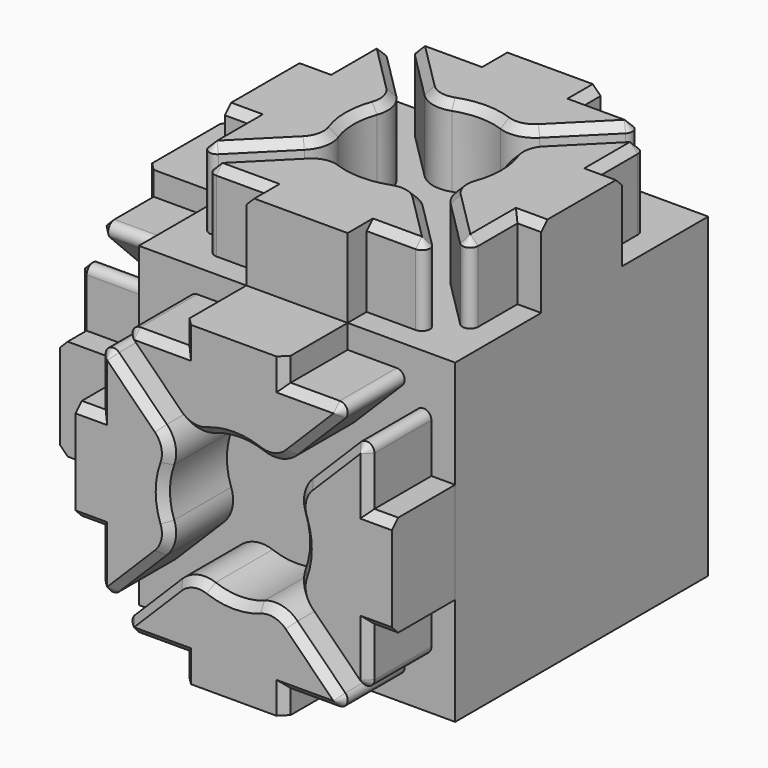
from build123d import *

# Parameters (mm, degrees)
F1_DEPTH     = 5
F3_DEPTH     = 5
F5_DEPTH     = 5
F6_R         = 2.5
F7_DEPTH     = 20
F8_T1_DEPTH  = 8.0177669558
F8_T3_DEPTH  = 8.0177669501
F8_T5_DEPTH  = 8.017766953
F8_T7_DEPTH  = 8.0177669501
F8_T9_DEPTH  = 8.0177669558
F8_T11_DEPTH = 8.0177655359
F8_T13_DEPTH = 8.01776837
F9_R         = 2
F10_SIZE     = 0.49999


# Not quite as in the source:
# - a fillet or chamfer that OpenCascade refuses, or shapes differently, is made with other operations: its cross-section is extruded or revolved along the edge and cut away or added
# - a fillet or chamfer is up to 0.001 mm smaller than in the source, because OpenCascade refuses the exact size


with BuildPart() as f1:
    # F0 (on Top) → F1 (new body)
    with BuildSketch(Plane.XY):
        with BuildLine():
            Line((13.2, 20), (6.8, 20))
            Line((6.8, 20), (6.8, 18.5))
            Line((6.8, 18.5), (2.4899494937, 18.5))
            Line((2.4899494937, 18.5), (7.3899494937, 13.6))
            ThreePointArc((7.3899494937, 13.6), (10, 14.4342618268), (12.6100505063, 13.6))
            Line((12.6100505063, 13.6), (17.5100505063, 18.5))
            Line((17.5100505063, 18.5), (13.2, 18.5))
            Line((13.2, 18.5), (13.2, 20))
        make_face()
    extrude(amount=F1_DEPTH)



with BuildPart() as f1b:
    # F0 (on Top) → F1, piece 2 (new body)
    with BuildSketch(Plane.XY):
        with BuildLine():
            Line((18.5, 6.8), (20, 6.8))
            Line((20, 6.8), (20, 13.2))
            Line((20, 13.2), (18.5, 13.2))
            Line((18.5, 13.2), (18.5, 17.5100505063))
            Line((18.5, 17.5100505063), (13.6, 12.6100505063))
            ThreePointArc((13.6, 12.6100505063), (14.4342618268, 10), (13.6, 7.3899494937))
            Line((13.6, 7.3899494937), (18.5, 2.4899494937))
            Line((18.5, 2.4899494937), (18.5, 6.8))
        make_face()
    extrude(amount=F1_DEPTH)


with BuildPart() as f1c:
    # F0 (on Top) → F1, piece 3 (new body)
    with BuildSketch(Plane.XY):
        with BuildLine():
            Line((6.8, 1.5), (6.8, 0))
            Line((6.8, 0), (13.2, 0))
            Line((13.2, 0), (13.2, 1.5))
            Line((13.2, 1.5), (17.5100505063, 1.5))
            Line((17.5100505063, 1.5), (12.6100505063, 6.4))
            ThreePointArc((12.6100505063, 6.4), (10, 5.5657381732), (7.3899494937, 6.4))
            Line((7.3899494937, 6.4), (2.4899494937, 1.5))
            Line((2.4899494937, 1.5), (6.8, 1.5))
        make_face()
    extrude(amount=F1_DEPTH)

    # F4 (on Front) → F5 (join)
    with BuildSketch(Plane.XZ):
        with BuildLine():
            Line((2.4899494963, -1.5), (7.3899494979, -6.3999999951))
            ThreePointArc((7.3899494979, -6.3999999951), (9.9999827045, -5.5657504858), (12.6100159112, -6.3999999951))
            Line((12.6100159112, -6.3999999951), (17.5100159046, -1.4999999951))
            Line((17.5100159046, -1.4999999951), (13.1999827087, -1.4999999951))
            Line((13.1999827087, -1.4999999951), (13.1999827087, 0))
            Line((13.1999827087, 0), (6.7999827087, 0))
            Line((6.7999827087, 0), (6.7999827087, -1.5))
            Line((6.7999827087, -1.5), (2.4899494963, -1.5))
        make_face()
    extrude(amount=F5_DEPTH)


with BuildPart() as f1d:
    # F0 (on Top) → F1, piece 4 (new body)
    with BuildSketch(Plane.XY):
        with BuildLine():
            Line((1.5, 6.8), (1.5, 2.4899494937))
            Line((1.5, 2.4899494937), (6.4, 7.3899494937))
            ThreePointArc((6.4, 7.3899494937), (5.5657381732, 10), (6.4, 12.6100505063))
            Line((6.4, 12.6100505063), (1.5, 17.5100505063))
            Line((1.5, 17.5100505063), (1.5, 13.2))
            Line((1.5, 13.2), (0, 13.2))
            Line((0, 13.2), (0, 6.8))
            Line((0, 6.8), (1.5, 6.8))
        make_face()
    extrude(amount=F1_DEPTH)

    # F2 (on Right) → F3 (join)
    with BuildSketch(Plane.YZ):
        with BuildLine():
            Line((2.4899734284, -1.5000000049), (7.38997343, -6.4))
            ThreePointArc((7.38997343, -6.4), (10.0000066366, -5.5657504907), (12.6100398432, -6.4))
            Line((12.6100398432, -6.4), (17.5100398367, -1.5))
            Line((17.5100398367, -1.5), (13.1999893277, -1.5))
            Line((13.1999893277, -1.5), (13.1999893277, -4.9e-09))
            Line((13.1999893277, -4.9e-09), (6.8000066408, -4.9e-09))
            Line((6.8000066408, -4.9e-09), (6.8000066408, -1.5000000049))
            Line((6.8000066408, -1.5000000049), (2.4899734284, -1.5000000049))
        make_face()
    extrude(amount=-F3_DEPTH)


with BuildPart() as f3:
    # F2 (on Right) → F3, piece 2 (new body)
    with BuildSketch(Plane.YZ):
        with BuildLine():
            Line((18.5000132602, -2.4899255639), (13.5999893277, -7.3899495029))
            ThreePointArc((13.5999893277, -7.3899495029), (14.4342388275, -9.9999826961), (13.5999893277, -12.6100158894))
            Line((13.5999893277, -12.6100158894), (18.4999893277, -17.5100158829))
            Line((18.4999893277, -17.5100158829), (18.4999893277, -13.1999827003))
            Line((18.4999893277, -13.1999827003), (20.0000066408, -13.1999827003))
            Line((20.0000066408, -13.1999827003), (20.0000132601, -6.8))
            Line((20.0000132601, -6.8), (18.5000132602, -6.8))
            Line((18.5000132602, -6.8), (18.5000132602, -2.4899255639))
        make_face()
    extrude(amount=-F3_DEPTH)


with BuildPart() as f3b:
    # F2 (on Right) → F3, piece 3 (new body)
    with BuildSketch(Plane.YZ):
        with BuildLine():
            ThreePointArc((12.6100571512, -13.5999827003), (10.0000059036, -14.4342445286), (7.38995493, -13.5999818427))
            Line((7.38995493, -13.5999818427), (2.4899499917, -18.499983527))
            Line((2.4899499917, -18.499983527), (6.8000004981, -18.499983527))
            Line((6.8000004981, -18.499983527), (6.8000004981, -19.999983527))
            Line((6.8000004981, -19.999983527), (13.2000004981, -19.9999835137))
            Line((13.2000004981, -19.9999835137), (13.2000004981, -18.4999827003))
            Line((13.2000004981, -18.4999827003), (17.5100571578, -18.4999827003))
            Line((17.5100571578, -18.4999827003), (12.6100571512, -13.5999827003))
        make_face()
    extrude(amount=-F3_DEPTH)


with BuildPart() as f3c:
    # F2 (on Right) → F3, piece 4 (new body)
    with BuildSketch(Plane.YZ):
        with BuildLine():
            Line((1.5000008268, -13.1999827003), (1.5000008268, -17.5100337047))
            Line((1.5000008268, -17.5100337047), (6.4000024537, -12.6100353317))
            ThreePointArc((6.4000024537, -12.6100353317), (5.5657406284, -9.9999825644), (6.4000050789, -7.3899306362))
            Line((6.4000050789, -7.3899306362), (1.5, -2.4899255639))
            Line((1.5, -2.4899255639), (1.5, -6.7999827003))
            Line((1.5, -6.7999827003), (0, -6.7999827003))
            Line((0, -6.7999827003), (6.6408e-06, -13.1999827003))
            Line((6.6408e-06, -13.1999827003), (1.5000008268, -13.1999827003))
        make_face()
    extrude(amount=-F3_DEPTH)

    # F4 (on Front) → F5, piece 4 (join)
    with BuildSketch(Plane.XZ):
        with BuildLine():
            Line((1.4999827087, -13.1999826954), (1.4999827087, -17.5100332017))
            Line((1.4999827087, -17.5100332017), (6.3999827087, -12.6100332017))
            ThreePointArc((6.3999827087, -12.6100332017), (5.5657208833, -9.9999826974), (6.3999827087, -7.3899321932))
            Line((6.3999827087, -7.3899321932), (1.4999760679, -2.4899255589))
            Line((1.4999760679, -2.4899255589), (1.4999760679, -6.7999826954))
            Line((1.4999760679, -6.7999826954), (-2.39321e-05, -6.7999826954))
            Line((-2.39321e-05, -6.7999826954), (-1.72913e-05, -13.1999826954))
            Line((-1.72913e-05, -13.1999826954), (1.4999827087, -13.1999826954))
        make_face()
    extrude(amount=F5_DEPTH)


with BuildPart() as f5:
    # F4 (on Front) → F5, piece 2 (new body)
    with BuildSketch(Plane.XZ):
        with BuildLine():
            Line((18.4999893281, -2.4899255589), (13.5999653956, -7.3899494979))
            ThreePointArc((13.5999653956, -7.3899494979), (14.4342148954, -9.9999826912), (13.5999653956, -12.6100158845))
            Line((13.5999653956, -12.6100158845), (18.4999653956, -17.510015878))
            Line((18.4999653956, -17.510015878), (18.4999653956, -13.1999826954))
            Line((18.4999653956, -13.1999826954), (19.9999827087, -13.1999826954))
            Line((19.9999827087, -13.1999826954), (19.9999893281, -6.7999826954))
            Line((19.9999893281, -6.7999826954), (18.4999893281, -6.7999826954))
            Line((18.4999893281, -6.7999826954), (18.4999893281, -2.4899255589))
        make_face()
    extrude(amount=F5_DEPTH)


with BuildPart() as f5b:
    # F4 (on Front) → F5, piece 3 (new body)
    with BuildSketch(Plane.XZ):
        with BuildLine():
            ThreePointArc((12.6100332192, -13.5999826954), (9.9999827108, -14.4342445236), (7.3899322023, -13.5999826954))
            Line((7.3899322023, -13.5999826954), (2.4899322023, -18.4999826954))
            Line((2.4899322023, -18.4999826954), (6.7999827087, -18.4999826954))
            Line((6.7999827087, -18.4999826954), (6.7999827087, -19.9999826954))
            Line((6.7999827087, -19.9999826954), (13.1999827087, -19.999982682))
            Line((13.1999827087, -19.999982682), (13.1999827087, -18.4999826954))
            Line((13.1999827087, -18.4999826954), (17.5100332257, -18.4999826954))
            Line((17.5100332257, -18.4999826954), (12.6100332192, -13.5999826954))
        make_face()
    extrude(amount=F5_DEPTH)


with BuildPart() as f1_1:
    add(f1.part)

    add(f1b.part)  # F7 merges F1b

    add(f1c.part)  # F7 merges F1c

    add(f1d.part)  # F7 merges F1d

    add(f3.part)  # F7 merges F3

    add(f3b.part)  # F7 merges F3b

    add(f3c.part)  # F7 merges F3c

    add(f5.part)  # F7 merges F5

    add(f5b.part)  # F7 merges F5b
    # F6 (on face) → F7 (join)
    with BuildSketch(Plane.XY):
        with BuildLine():
            Line((0, 6.8), (0, 0))
            Line((0, 0), (6.8, 0))
            Line((6.8, 0), (6.8, 1.5))
            Line((6.8, 1.5), (2.4899494937, 1.5))
            Line((2.4899494937, 1.5), (7.3899494937, 6.4))
            ThreePointArc((7.3899494937, 6.4), (10, 5.5657381732), (12.6100505063, 6.4))
            Line((12.6100505063, 6.4), (17.5100505063, 1.5))
            Line((17.5100505063, 1.5), (13.2, 1.5))
            Line((13.2, 1.5), (13.2, 0))
            Line((13.2, 0), (20, 0))
            Line((20, 0), (20, 6.8))
            Line((20, 6.8), (18.5, 6.8))
            Line((18.5, 6.8), (18.5, 2.4899494937))
            Line((18.5, 2.4899494937), (13.6, 7.3899494937))
            ThreePointArc((13.6, 7.3899494937), (14.4342618268, 10), (13.6, 12.6100505063))
            Line((13.6, 12.6100505063), (18.5, 17.5100505063))
            Line((18.5, 17.5100505063), (18.5, 13.2))
            Line((18.5, 13.2), (20, 13.2))
            Line((20, 13.2), (20, 20))
            Line((20, 20), (13.2, 20))
            Line((13.2, 20), (13.2, 18.5))
            Line((13.2, 18.5), (17.5100505063, 18.5))
            Line((17.5100505063, 18.5), (12.6100505063, 13.6))
            ThreePointArc((12.6100505063, 13.6), (10, 14.4342618268), (7.3899494937, 13.6))
            Line((7.3899494937, 13.6), (2.4899494937, 18.5))
            Line((2.4899494937, 18.5), (6.8, 18.5))
            Line((6.8, 18.5), (6.8, 20))
            Line((6.8, 20), (0, 20))
            Line((0, 20), (0, 13.2))
            Line((0, 13.2), (1.5, 13.2))
            Line((1.5, 13.2), (1.5, 17.5100505063))
            Line((1.5, 17.5100505063), (6.4, 12.6100505063))
            ThreePointArc((6.4, 12.6100505063), (5.5657381732, 10), (6.4, 7.3899494937))
            Line((6.4, 7.3899494937), (1.5, 2.4899494937))
            Line((1.5, 2.4899494937), (1.5, 6.8))
            Line((1.5, 6.8), (0, 6.8))
        make_face()
        with Locations((10, 10)):
            Circle(F6_R, mode=Mode.SUBTRACT)
        with BuildLine():
            Line((18.5, 6.8), (20, 6.8))
            Line((20, 6.8), (20, 13.2))
            Line((20, 13.2), (18.5, 13.2))
            Line((18.5, 13.2), (18.5, 17.5100505063))
            Line((18.5, 17.5100505063), (13.6, 12.6100505063))
            ThreePointArc((13.6, 12.6100505063), (14.4342618268, 10), (13.6, 7.3899494937))
            Line((13.6, 7.3899494937), (18.5, 2.4899494937))
            Line((18.5, 2.4899494937), (18.5, 6.8))
        make_face()
        with BuildLine():
            Line((13.2, 20), (6.8, 20))
            Line((6.8, 20), (6.8, 18.5))
            Line((6.8, 18.5), (2.4899494937, 18.5))
            Line((2.4899494937, 18.5), (7.3899494937, 13.6))
            ThreePointArc((7.3899494937, 13.6), (10, 14.4342618268), (12.6100505063, 13.6))
            Line((12.6100505063, 13.6), (17.5100505063, 18.5))
            Line((17.5100505063, 18.5), (13.2, 18.5))
            Line((13.2, 18.5), (13.2, 20))
        make_face()
        with BuildLine():
            Line((0, 13.2), (0, 6.8))
            Line((0, 6.8), (1.5, 6.8))
            Line((1.5, 6.8), (1.5, 2.4899494937))
            Line((1.5, 2.4899494937), (6.4, 7.3899494937))
            ThreePointArc((6.4, 7.3899494937), (5.5657381732, 10), (6.4, 12.6100505063))
            Line((6.4, 12.6100505063), (1.5, 17.5100505063))
            Line((1.5, 17.5100505063), (1.5, 13.2))
            Line((1.5, 13.2), (0, 13.2))
        make_face()
        with BuildLine():
            Line((6.8, 1.5), (6.8, 0))
            Line((6.8, 0), (13.2, 0))
            Line((13.2, 0), (13.2, 1.5))
            Line((13.2, 1.5), (17.5100505063, 1.5))
            Line((17.5100505063, 1.5), (12.6100505063, 6.4))
            ThreePointArc((12.6100505063, 6.4), (10, 5.5657381732), (7.3899494937, 6.4))
            Line((7.3899494937, 6.4), (2.4899494937, 1.5))
            Line((2.4899494937, 1.5), (6.8, 1.5))
        make_face()
        with Locations((10, 10)):
            Circle(F6_R)
    extrude(amount=-F7_DEPTH)

    # F8: fillet of radius 0.5 on 24 edges, made by hand

    # F8_s2 → F8_t1 (cut)
    with BuildSketch(Plane.XZ):
        with BuildLine():
            ThreePointArc((18.4999893281, -3.6970323413), (18.1913310441, -3.2350925749), (17.6464359373, -3.3434789509))
            Line((17.6464359373, -3.3434789509), (18.4999893281, -2.4899255589))
            Line((18.4999893281, -2.4899255589), (18.4999893281, -3.6970323413))
        make_face()
        with BuildLine():
            ThreePointArc((16.3029264434, -18.4999826954), (16.7648662097, -18.1913244114), (16.6564798337, -17.6464293045))
            Line((16.6564798337, -17.6464293045), (17.5100332257, -18.4999826954))
            Line((17.5100332257, -18.4999826954), (16.3029264434, -18.4999826954))
        make_face()
        with BuildLine():
            ThreePointArc((3.6970562786, -1.5), (3.2351165123, -1.808658284), (3.3435028883, -2.3535533908))
            Line((3.3435028883, -2.3535533908), (2.4899494963, -1.5))
            Line((2.4899494963, -1.5), (3.6970562786, -1.5))
        make_face()
    extrude(amount=F8_T1_DEPTH, mode=Mode.SUBTRACT)

    # F8_s4 → F8_t3 (cut)
    with BuildSketch(Plane.XZ):
        with BuildLine():
            ThreePointArc((16.6564625154, -2.3535533854), (16.7648488908, -1.8086582787), (16.3029091246, -1.4999999951))
            Line((16.3029091246, -1.4999999951), (17.5100159046, -1.4999999951))
            Line((17.5100159046, -1.4999999951), (16.6564625154, -2.3535533854))
        make_face()
        with BuildLine():
            ThreePointArc((18.4999653956, -16.3029090979), (18.191307112, -16.7648488641), (17.6464120053, -16.6564624887))
            Line((17.6464120053, -16.6564624887), (18.4999653956, -17.510015878))
            Line((18.4999653956, -17.510015878), (18.4999653956, -16.3029090979))
        make_face()
        with BuildLine():
            ThreePointArc((3.3434855929, -17.6464293048), (3.2350992173, -18.1913244115), (3.6970389835, -18.4999826954))
            Line((3.6970389835, -18.4999826954), (2.4899322023, -18.4999826954))
            Line((2.4899322023, -18.4999826954), (3.3434855929, -17.6464293048))
        make_face()
        with BuildLine():
            ThreePointArc((2.3535360993, -16.6564798111), (1.8086409925, -16.7648661868), (1.4999827087, -16.3029264205))
            Line((1.4999827087, -16.3029264205), (1.4999827087, -17.5100332017))
            Line((1.4999827087, -17.5100332017), (2.3535360993, -16.6564798111))
        make_face()
        with BuildLine():
            ThreePointArc((1.4999760679, -3.697032339), (1.8086343516, -3.2350925728), (2.3535294583, -3.3434789482))
            Line((2.3535294583, -3.3434789482), (1.4999760679, -2.4899255589))
            Line((1.4999760679, -2.4899255589), (1.4999760679, -3.697032339))
        make_face()
    extrude(amount=F8_T3_DEPTH, mode=Mode.SUBTRACT)

    # F8_s6 → F8_t5 (cut)
    with BuildSketch(Plane.XY):
        with BuildLine():
            ThreePointArc((3.3435028843, 2.3535533906), (3.2351165086, 1.8086582838), (3.6970562748, 1.5))
            Line((3.6970562748, 1.5), (2.4899494937, 1.5))
            Line((2.4899494937, 1.5), (3.3435028843, 2.3535533906))
        make_face()
        with BuildLine():
            ThreePointArc((1.5, 3.6970562748), (1.8086582838, 3.2351165086), (2.3535533906, 3.3435028843))
            Line((2.3535533906, 3.3435028843), (1.5, 2.4899494937))
            Line((1.5, 2.4899494937), (1.5, 3.6970562748))
        make_face()
        with BuildLine():
            ThreePointArc((16.3029437252, 1.5), (16.7648834914, 1.8086582838), (16.6564971157, 2.3535533906))
            Line((16.6564971157, 2.3535533906), (17.5100505063, 1.5))
            Line((17.5100505063, 1.5), (16.3029437252, 1.5))
        make_face()
        with BuildLine():
            ThreePointArc((17.6464466094, 3.3435028843), (18.1913417162, 3.2351165086), (18.5, 3.6970562748))
            Line((18.5, 3.6970562748), (18.5, 2.4899494937))
            Line((18.5, 2.4899494937), (17.6464466094, 3.3435028843))
        make_face()
        with BuildLine():
            ThreePointArc((18.5, 16.3029437252), (18.1913417162, 16.7648834914), (17.6464466094, 16.6564971157))
            Line((17.6464466094, 16.6564971157), (18.5, 17.5100505063))
            Line((18.5, 17.5100505063), (18.5, 16.3029437252))
        make_face()
        with BuildLine():
            ThreePointArc((16.6564971157, 17.6464466094), (16.7648834914, 18.1913417162), (16.3029437252, 18.5))
            Line((16.3029437252, 18.5), (17.5100505063, 18.5))
            Line((17.5100505063, 18.5), (16.6564971157, 17.6464466094))
        make_face()
        with BuildLine():
            ThreePointArc((3.6970562748, 18.5), (3.2351165086, 18.1913417162), (3.3435028843, 17.6464466094))
            Line((3.3435028843, 17.6464466094), (2.4899494937, 18.5))
            Line((2.4899494937, 18.5), (3.6970562748, 18.5))
        make_face()
        with BuildLine():
            ThreePointArc((2.3535533906, 16.6564971157), (1.8086582838, 16.7648834914), (1.5, 16.3029437252))
            Line((1.5, 16.3029437252), (1.5, 17.5100505063))
            Line((1.5, 17.5100505063), (2.3535533906, 16.6564971157))
        make_face()
    extrude(amount=F8_T5_DEPTH, mode=Mode.SUBTRACT)

    # F8_s8 → F8_t7 (cut)
    with BuildSketch(Plane.YZ.offset(-8.0177669501)):
        with BuildLine():
            ThreePointArc((16.3029330567, -1.5), (16.7648728228, -1.8086582837), (16.6564864475, -2.3535533904))
            Line((16.6564864475, -2.3535533904), (17.5100398367, -1.5))
            Line((17.5100398367, -1.5), (16.3029330567, -1.5))
        make_face()
        with BuildLine():
            ThreePointArc((1.5, -3.6970323439), (1.8086582837, -3.2350925777), (2.3535533904, -3.3434789531))
            Line((2.3535533904, -3.3434789531), (1.5, -2.4899255639))
            Line((1.5, -2.4899255639), (1.5, -3.6970323439))
        make_face()
        with BuildLine():
            ThreePointArc((18.4999893277, -16.3029091028), (18.191331044, -16.764848869), (17.6464359373, -16.6564624937))
            Line((17.6464359373, -16.6564624937), (18.4999893277, -17.5100158829))
            Line((18.4999893277, -17.5100158829), (18.4999893277, -16.3029091028))
        make_face()
    extrude(amount=F8_T7_DEPTH, mode=Mode.SUBTRACT)

    # F8_s10 → F8_t9 (cut)
    with BuildSketch(Plane.YZ.offset(-8.0177669558)):
        with BuildLine():
            ThreePointArc((17.6464598693, -3.3434789558), (18.1913549762, -3.2350925799), (18.5000132602, -3.6970323462))
            Line((18.5000132602, -3.6970323462), (18.5000132602, -2.4899255639))
            Line((18.5000132602, -2.4899255639), (17.6464598693, -3.3434789558))
        make_face()
        with BuildLine():
            ThreePointArc((3.6970802107, -1.5000000049), (3.2351404444, -1.8086582889), (3.3435268204, -2.3535533958))
            Line((3.3435268204, -2.3535533958), (2.4899734284, -1.5000000049))
            Line((2.4899734284, -1.5000000049), (3.6970802107, -1.5000000049))
        make_face()
        with BuildLine():
            ThreePointArc((16.6565037658, -17.6464293095), (16.7648901418, -18.1913244163), (16.3029503754, -18.4999827003))
            Line((16.3029503754, -18.4999827003), (17.5100571578, -18.4999827003))
            Line((17.5100571578, -18.4999827003), (16.6565037658, -17.6464293095))
        make_face()
    extrude(amount=F8_T9_DEPTH, mode=Mode.SUBTRACT)

    # F8_s12 → F8_t11 (cut)
    with BuildSketch(Plane.YZ.offset(-8.0177655359)):
        with BuildLine():
            ThreePointArc((2.3535541, -16.6564809983), (1.8086590339, -16.7648672248), (1.5000008268, -16.3029274903))
            Line((1.5000008268, -16.3029274903), (1.5000008268, -17.5100337047))
            Line((1.5000008268, -17.5100337047), (2.3535541, -16.6564809983))
        make_face()
    extrude(amount=F8_T11_DEPTH, mode=Mode.SUBTRACT)

    # F8_s14 → F8_t13 (cut)
    with BuildSketch(Plane.YZ.offset(-8.01776837)):
        with BuildLine():
            ThreePointArc((3.3435040665, -17.6464300191), (3.2351175417, -18.1913251665), (3.6970573397, -18.499983527))
            Line((3.6970573397, -18.499983527), (2.4899499917, -18.499983527))
            Line((2.4899499917, -18.499983527), (3.3435040665, -17.6464300191))
        make_face()
    extrude(amount=F8_T13_DEPTH, mode=Mode.SUBTRACT)

    # F9 (call 1 of 24: OpenCascade refuses the feature's edges together)
    f9_edges = [f1_1.edges().sort_by_distance(p)[0] for p in [
        (-2.5, 13.599989, -7.38995),
    ]]
    fillet(f9_edges, radius=F9_R)

    # F9#2 (call 2 of 24)
    f9_2_edges = [f1_1.edges().sort_by_distance(p)[0] for p in [
        (-2.5, 13.599989, -12.610016),
    ]]
    fillet(f9_2_edges, radius=F9_R)

    # F9#3 (call 3 of 24)
    f9_3_edges = [f1_1.edges().sort_by_distance(p)[0] for p in [
        (-2.5, 12.61004, -6.4),
    ]]
    fillet(f9_3_edges, radius=F9_R)

    # F9#4 (call 4 of 24)
    f9_4_edges = [f1_1.edges().sort_by_distance(p)[0] for p in [
        (-2.5, 7.389973, -6.4),
    ]]
    fillet(f9_4_edges, radius=F9_R)

    # F9#5 (call 5 of 24)
    f9_5_edges = [f1_1.edges().sort_by_distance(p)[0] for p in [
        (-2.5, 6.400002, -12.610035),
    ]]
    fillet(f9_5_edges, radius=F9_R)

    # F9#6 (call 6 of 24)
    f9_6_edges = [f1_1.edges().sort_by_distance(p)[0] for p in [
        (-2.5, 6.400005, -7.389931),
    ]]
    fillet(f9_6_edges, radius=F9_R)

    # F9#7 (call 7 of 24)
    f9_7_edges = [f1_1.edges().sort_by_distance(p)[0] for p in [
        (-2.5, 12.610057, -13.599983),
    ]]
    fillet(f9_7_edges, radius=F9_R)

    # F9#8 (call 8 of 24)
    f9_8_edges = [f1_1.edges().sort_by_distance(p)[0] for p in [
        (-2.5, 7.389955, -13.599982),
    ]]
    fillet(f9_8_edges, radius=F9_R)

    # F9#9 (call 9 of 24)
    f9_9_edges = [f1_1.edges().sort_by_distance(p)[0] for p in [
        (6.399983, -2.5, -7.389932),
    ]]
    fillet(f9_9_edges, radius=F9_R)

    # F9#10 (call 10 of 24)
    f9_10_edges = [f1_1.edges().sort_by_distance(p)[0] for p in [
        (6.399983, -2.5, -12.610033),
    ]]
    fillet(f9_10_edges, radius=F9_R)

    # F9#11 (call 11 of 24)
    f9_11_edges = [f1_1.edges().sort_by_distance(p)[0] for p in [
        (7.389932, -2.5, -13.599983),
    ]]
    fillet(f9_11_edges, radius=F9_R)

    # F9#12 (call 12 of 24)
    f9_12_edges = [f1_1.edges().sort_by_distance(p)[0] for p in [
        (12.610033, -2.5, -13.599983),
    ]]
    fillet(f9_12_edges, radius=F9_R)

    # F9#13 (call 13 of 24)
    f9_13_edges = [f1_1.edges().sort_by_distance(p)[0] for p in [
        (13.599965, -2.5, -12.610016),
    ]]
    fillet(f9_13_edges, radius=F9_R)

    # F9#14 (call 14 of 24)
    f9_14_edges = [f1_1.edges().sort_by_distance(p)[0] for p in [
        (7.389949, -2.5, -6.4),
    ]]
    fillet(f9_14_edges, radius=F9_R)

    # F9#15 (call 15 of 24)
    f9_15_edges = [f1_1.edges().sort_by_distance(p)[0] for p in [
        (12.610016, -2.5, -6.4),
    ]]
    fillet(f9_15_edges, radius=F9_R)

    # F9#16 (call 16 of 24)
    f9_16_edges = [f1_1.edges().sort_by_distance(p)[0] for p in [
        (13.599965, -2.5, -7.389949),
    ]]
    fillet(f9_16_edges, radius=F9_R)

    # F9#17 (call 17 of 24)
    f9_17_edges = [f1_1.edges().sort_by_distance(p)[0] for p in [
        (6.4, 12.610051, 2.5),
    ]]
    fillet(f9_17_edges, radius=F9_R)

    # F9#18 (call 18 of 24)
    f9_18_edges = [f1_1.edges().sort_by_distance(p)[0] for p in [
        (6.4, 7.389949, 2.5),
    ]]
    fillet(f9_18_edges, radius=F9_R)

    # F9#19 (call 19 of 24)
    f9_19_edges = [f1_1.edges().sort_by_distance(p)[0] for p in [
        (7.389949, 6.4, 2.5),
    ]]
    fillet(f9_19_edges, radius=F9_R)

    # F9#20 (call 20 of 24)
    f9_20_edges = [f1_1.edges().sort_by_distance(p)[0] for p in [
        (13.6, 7.389949, 2.5),
    ]]
    fillet(f9_20_edges, radius=F9_R)

    # F9#21 (call 21 of 24)
    f9_21_edges = [f1_1.edges().sort_by_distance(p)[0] for p in [
        (12.610051, 6.4, 2.5),
    ]]
    fillet(f9_21_edges, radius=F9_R)

    # F9#22 (call 22 of 24)
    f9_22_edges = [f1_1.edges().sort_by_distance(p)[0] for p in [
        (12.610051, 13.6, 2.5),
    ]]
    fillet(f9_22_edges, radius=F9_R)

    # F9#23 (call 23 of 24)
    f9_23_edges = [f1_1.edges().sort_by_distance(p)[0] for p in [
        (7.389949, 13.6, 2.5),
    ]]
    fillet(f9_23_edges, radius=F9_R)

    # F9#24 (call 24 of 24)
    f9_24_edges = [f1_1.edges().sort_by_distance(p)[0] for p in [
        (13.6, 12.610051, 2.5),
    ]]
    fillet(f9_24_edges, radius=F9_R)

    # F10 (size 0.5 in the source; OpenCascade refuses exactly that, so slightly less here)
    f10_edges = [f1_1.edges().sort_by_distance(p)[0] for p in [
        (15.147161, -5, -3.862855),
        (13.199983, -5, -0.75),
        (6.799983, -5, -0.75),
        (14.089412, -5, -7.343525),
        (9.999983, -5, -14.434245),
        (6.799983, -5, -19.249983),
        (13.199983, -5, -19.249983),
        (19.249974, -5, -13.199983),
        (19.249989, -5, -6.799983),
        (5.565721, -5, -9.999983),
        (0.749976, -5, -6.799983),
        (0.749983, -5, -13.199983),
        (3.862852, 4.852802, 5),
        (10, 14.434262, 5),
        (14.434262, 10, 5),
        (10, 5.565738, 5),
        (19.25, 6.8, 5),
        (0.75, 6.8, 5),
        (13.2, 19.25, 5),
        (6.8, 19.25, 5),
        (6.8, 0.75, 5),
        (0.75, 13.2, 5),
        (-5, 10.000006, -14.434245),
        (-5, 14.434239, -9.999983),
        (-5, 10.000007, -5.56575),
        (-5, 5.565741, -9.999983),
        (-5, 19.249998, -13.199983),
        (-5, 13.2, -19.249983),
        (-5, 0.750004, -13.199983),
        (-5, 13.199989, -0.75),
        (-5, 6.800007, -0.75),
        (-5, 6.8, -19.249984),
        (-5, 0.75, -6.799983),
        (-5, 19.250013, -6.8),
        (19.25, 13.2, 5),
        (16.137148, 15.147198, 5),
        (14.08945, 12.656476, 5),
        (18.191342, 16.764883, 5),
        (18.5, 14.751472, 5),
        (14.08945, 7.343524, 5),
        (16.137148, 4.852802, 5),
        (18.191342, 3.235117, 5),
        (18.5, 5.248528, 5),
        (14.751472, 18.5, 5),
        (16.764883, 18.191342, 5),
        (15.147198, 16.137148, 5),
        (12.656476, 14.08945, 5),
        (14.751472, 1.5, 5),
        (16.764883, 1.808658, 5),
        (7.343524, 14.08945, 5),
        (15.147198, 3.862852, 5),
        (4.852802, 16.137148, 5),
        (12.656476, 5.91055, 5),
        (3.235117, 18.191342, 5),
        (5.248528, 18.5, 5),
        (7.343524, 5.91055, 5),
        (4.852802, 3.862852, 5),
        (3.235117, 1.808658, 5),
        (5.248528, 1.5, 5),
        (1.5, 14.751472, 5),
        (1.808658, 16.764883, 5),
        (3.862852, 15.147198, 5),
        (9.999983, -5, -5.56575),
        (12.65644, -5, -5.910553),
        (7.343525, -5, -5.910553),
        (4.852804, -5, -3.862855),
        (16.764849, -5, -1.808658),
        (3.235117, -5, -1.808658),
        (14.751446, -5, -1.5),
        (5.248519, -5, -1.5),
        (5.91055, 12.656476, 5),
        (5.565738, 10, 5),
        (5.91055, 7.343524, 5),
        (1.808658, 3.235117, 5),
        (1.5, 5.248528, 5),
        (14.434215, -5, -9.999983),
        (14.089412, -5, -12.65644),
        (16.137123, -5, -4.852792),
        (16.137111, -5, -15.147161),
        (18.191331, -5, -3.235093),
        (18.191307, -5, -16.764849),
        (18.499989, -5, -5.248508),
        (18.499965, -5, -14.751446),
        (1.499976, -5, -5.248508),
        (1.808634, -5, -3.235093),
        (3.862832, -5, -4.852781),
        (5.910532, -5, -7.343507),
        (5.910532, -5, -12.656459),
        (1.499983, -5, -14.751455),
        (3.862835, -5, -15.147181),
        (1.808641, -5, -16.764866),
        (12.656459, -5, -14.089433),
        (7.343507, -5, -14.089433),
        (15.147181, -5, -16.13713),
        (4.852785, -5, -16.13713),
        (16.764866, -5, -18.191324),
        (3.235099, -5, -18.191324),
        (14.751455, -5, -18.499983),
        (5.248511, -5, -18.499983),
        (-5, 7.343529, -14.089432),
        (-5, 12.656483, -14.089433),
        (-5, 4.852805, -16.13713),
        (-5, 15.147205, -16.13713),
        (-5, 3.235118, -18.191325),
        (-5, 16.76489, -18.191324),
        (-5, 5.248529, -18.499984),
        (-5, 14.751475, -18.499983),
        (-5, 5.910554, -7.343505),
        (-5, 5.910552, -12.656461),
        (-5, 3.862855, -4.85278),
        (-5, 3.862854, -15.147182),
        (-5, 1.808658, -3.235093),
        (-5, 1.808659, -16.764867),
        (-5, 1.5, -5.248508),
        (-5, 1.500001, -14.751455),
        (-5, 7.343549, -5.910553),
        (-5, 12.656464, -5.910553),
        (-5, 4.852828, -3.862855),
        (-5, 15.147185, -3.862855),
        (-5, 3.23514, -1.808658),
        (-5, 16.764873, -1.808658),
        (-5, 5.248543, -1.5),
        (-5, 14.751461, -1.5),
        (-5, 14.089436, -12.65644),
        (-5, 14.089436, -7.343525),
        (-5, 16.137135, -15.147161),
        (-5, 16.137147, -4.852792),
        (-5, 18.191331, -16.764849),
        (-5, 18.191355, -3.235093),
        (-5, 18.499989, -14.751446),
        (-5, 18.500013, -5.248516),
    ]]
    chamfer(f10_edges, length=F10_SIZE)


solid = f1_1.part
